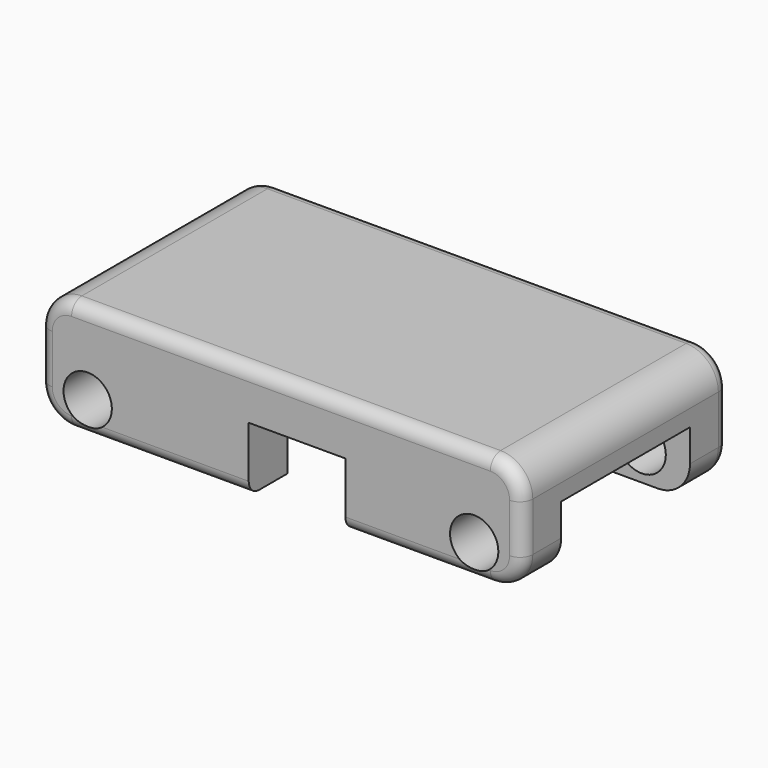
from build123d import *

# Parameters (mm, degrees)
F0_R          = 4.7625
F1_DEPTH      = 25.4
F2_W          = 31.75
F2_H          = 12.7
F3_DEPTH      = 47.626
F3_DEPTH_BACK = 47.626
F4_T1_DEPTH   = 82.55
F4_T3_DEPTH   = 9.6279704779
F4_T5_DEPTH   = 41.275
F4_T7_DEPTH   = 34.925
F4_T10_ANGLE  = 90
F4_T12_ANGLE  = 90
F4_T14_ANGLE  = 90
F4_T16_ANGLE  = 90
F4_T18_ANGLE  = 90
F4_T20_ANGLE  = 90
F4_T22_ANGLE  = 90
F4_T24_ANGLE  = 90


# Not quite as in the source:
# - a fillet or chamfer that OpenCascade refuses, or shapes differently, is made with other operations: its cross-section is extruded or revolved along the edge and cut away or added


with BuildPart() as f1:
    # F0 (on Front) → F1 (new body, symmetric)
    with BuildSketch(Plane.XZ):
        with BuildLine():
            Line((41.275, 15.9779704779), (-41.275, 15.9779704779))
            ThreePointArc((-41.275, 15.9779704779), (-45.7651280605, 14.1180985385), (-47.625, 9.6279704779))
            Line((-47.625, 9.6279704779), (-47.625, 0))
            ThreePointArc((-47.625, 0), (-45.7651280605, -4.4901280605), (-41.275, -6.35))
            Line((-41.275, -6.35), (-6.35, -6.35))
            Line((-6.35, -6.35), (-6.35, 6.35))
            Line((-6.35, 6.35), (12.7, 6.35))
            Line((12.7, 6.35), (12.7, -6.35))
            Line((12.7, -6.35), (41.275, -6.35))
            ThreePointArc((41.275, -6.35), (45.7651280605, -4.4901280605), (47.625, 0))
            Line((47.625, 0), (47.625, 9.6279704779))
            ThreePointArc((47.625, 9.6279704779), (45.7651280605, 14.1180985385), (41.275, 15.9779704779))
        make_face()
        with Locations((-38.1, 0)):
            Circle(F0_R, mode=Mode.SUBTRACT)
        with Locations((38.1, 0)):
            Circle(F0_R, mode=Mode.SUBTRACT)
    extrude(amount=F1_DEPTH, both=True)

    # F2 (on Right) → F3 (cut, two sides)
    with BuildSketch(Plane.YZ) as f3_sk:
        Rectangle(F2_W, F2_H)
    extrude(amount=F3_DEPTH, mode=Mode.SUBTRACT)
    extrude(f3_sk.sketch, amount=-F3_DEPTH_BACK, mode=Mode.SUBTRACT)

    # F4: fillet of radius 2.54 on 18 edges, made by hand

    # F4_s2 → F4_t1 (cut)
    with BuildSketch(Plane.YZ.offset(-41.275)):
        with BuildLine():
            ThreePointArc((22.86, 15.9779704779), (24.6560512242, 15.2340217022), (25.4, 13.4379704779))
            Line((25.4, 13.4379704779), (25.4, 15.9779704779))
            Line((25.4, 15.9779704779), (22.86, 15.9779704779))
        make_face()
        with BuildLine():
            ThreePointArc((-22.86, 15.9779704779), (-24.6560512242, 15.2340217022), (-25.4, 13.4379704779))
            Line((-25.4, 13.4379704779), (-25.4, 15.9779704779))
            Line((-25.4, 15.9779704779), (-22.86, 15.9779704779))
        make_face()
    extrude(amount=F4_T1_DEPTH, mode=Mode.SUBTRACT)

    # F4_s4 → F4_t3 (cut)
    with BuildSketch(Plane.XY):
        with BuildLine():
            ThreePointArc((-45.085, 25.4), (-46.8810512242, 24.6560512242), (-47.625, 22.86))
            Line((-47.625, 22.86), (-47.625, 25.4))
            Line((-47.625, 25.4), (-45.085, 25.4))
        make_face()
        with BuildLine():
            ThreePointArc((45.085, 25.4), (46.8810512242, 24.6560512242), (47.625, 22.86))
            Line((47.625, 22.86), (47.625, 25.4))
            Line((47.625, 25.4), (45.085, 25.4))
        make_face()
        with BuildLine():
            ThreePointArc((-45.085, -25.4), (-46.8810512242, -24.6560512242), (-47.625, -22.86))
            Line((-47.625, -22.86), (-47.625, -25.4))
            Line((-47.625, -25.4), (-45.085, -25.4))
        make_face()
        with BuildLine():
            ThreePointArc((45.085, -25.4), (46.8810512242, -24.6560512242), (47.625, -22.86))
            Line((47.625, -22.86), (47.625, -25.4))
            Line((47.625, -25.4), (45.085, -25.4))
        make_face()
    extrude(amount=F4_T3_DEPTH, mode=Mode.SUBTRACT)

    # F4_s6 → F4_t5 (cut)
    with BuildSketch(Plane.YZ.offset(-41.275)):
        with BuildLine():
            ThreePointArc((25.4, -3.81), (24.6560512242, -5.6060512242), (22.86, -6.35))
            Line((22.86, -6.35), (25.4, -6.35))
            Line((25.4, -6.35), (25.4, -3.81))
        make_face()
        with BuildLine():
            ThreePointArc((-25.4, -3.81), (-24.6560512242, -5.6060512242), (-22.86, -6.35))
            Line((-22.86, -6.35), (-25.4, -6.35))
            Line((-25.4, -6.35), (-25.4, -3.81))
        make_face()
    extrude(amount=F4_T5_DEPTH, mode=Mode.SUBTRACT)

    # F4_s8 → F4_t7 (cut)
    with BuildSketch(Plane.YZ.offset(6.35)):
        with BuildLine():
            ThreePointArc((25.4, -3.81), (24.6560512242, -5.6060512242), (22.86, -6.35))
            Line((22.86, -6.35), (25.4, -6.35))
            Line((25.4, -6.35), (25.4, -3.81))
        make_face()
        with BuildLine():
            ThreePointArc((-25.4, -3.81), (-24.6560512242, -5.6060512242), (-22.86, -6.35))
            Line((-22.86, -6.35), (-25.4, -6.35))
            Line((-25.4, -6.35), (-25.4, -3.81))
        make_face()
    extrude(amount=F4_T7_DEPTH, mode=Mode.SUBTRACT)

    # F4_s9 → F4_t10 (revolve, cut)
    with BuildSketch(Plane.YZ.offset(-41.275)):
        with BuildLine():
            ThreePointArc((25.4, 13.4379704779), (24.6560512242, 15.2340217022), (22.86, 15.9779704779))
            Line((22.86, 15.9779704779), (25.4, 15.9779704779))
            Line((25.4, 15.9779704779), (25.4, 13.4379704779))
        make_face()
    revolve(axis=Axis((-41.275, 25.4, 9.6279704779), (0, -1, 0)), revolution_arc=F4_T10_ANGLE, mode=Mode.SUBTRACT)

    # F4_s11 → F4_t12 (revolve, cut)
    with BuildSketch(Plane.XY):
        with BuildLine():
            ThreePointArc((-45.085, 25.4), (-46.8810512242, 24.6560512242), (-47.625, 22.86))
            Line((-47.625, 22.86), (-47.625, 25.4))
            Line((-47.625, 25.4), (-45.085, 25.4))
        make_face()
    revolve(axis=Axis((-41.275, 25.4, 0), (0, -1, 0)), revolution_arc=F4_T12_ANGLE, mode=Mode.SUBTRACT)

    # F4_s13 → F4_t14 (revolve, cut)
    with BuildSketch(Plane.YZ.offset(41.275)):
        with BuildLine():
            ThreePointArc((25.4, -3.81), (24.6560512242, -5.6060512242), (22.86, -6.35))
            Line((22.86, -6.35), (25.4, -6.35))
            Line((25.4, -6.35), (25.4, -3.81))
        make_face()
    revolve(axis=Axis((41.275, 25.4, 0), (0, -1, 0)), revolution_arc=F4_T14_ANGLE, mode=Mode.SUBTRACT)

    # F4_s15 → F4_t16 (revolve, cut)
    with BuildSketch(Plane.XY.offset(9.6279704779)):
        with BuildLine():
            ThreePointArc((45.085, 25.4), (46.8810512242, 24.6560512242), (47.625, 22.86))
            Line((47.625, 22.86), (47.625, 25.4))
            Line((47.625, 25.4), (45.085, 25.4))
        make_face()
    revolve(axis=Axis((41.275, 25.4, 9.6279704779), (0, -1, 0)), revolution_arc=F4_T16_ANGLE, mode=Mode.SUBTRACT)

    # F4_s17 → F4_t18 (revolve, cut)
    with BuildSketch(Plane.YZ.offset(-41.275)):
        with BuildLine():
            ThreePointArc((-22.86, 15.9779704779), (-24.6560512242, 15.2340217022), (-25.4, 13.4379704779))
            Line((-25.4, 13.4379704779), (-25.4, 15.9779704779))
            Line((-25.4, 15.9779704779), (-22.86, 15.9779704779))
        make_face()
    revolve(axis=Axis((-41.275, -25.4, 9.6279704779), (0, -1, 0)), revolution_arc=F4_T18_ANGLE, mode=Mode.SUBTRACT)

    # F4_s19 → F4_t20 (revolve, cut)
    with BuildSketch(Plane.XY):
        with BuildLine():
            ThreePointArc((-45.085, -25.4), (-46.8810512242, -24.6560512242), (-47.625, -22.86))
            Line((-47.625, -22.86), (-47.625, -25.4))
            Line((-47.625, -25.4), (-45.085, -25.4))
        make_face()
    revolve(axis=Axis((-41.275, -25.4, 0), (0, -1, 0)), revolution_arc=F4_T20_ANGLE, mode=Mode.SUBTRACT)

    # F4_s21 → F4_t22 (revolve, cut)
    with BuildSketch(Plane.YZ.offset(41.275)):
        with BuildLine():
            ThreePointArc((-25.4, -3.81), (-24.6560512242, -5.6060512242), (-22.86, -6.35))
            Line((-22.86, -6.35), (-25.4, -6.35))
            Line((-25.4, -6.35), (-25.4, -3.81))
        make_face()
    revolve(axis=Axis((41.275, -25.4, 0), (0, -1, 0)), revolution_arc=F4_T22_ANGLE, mode=Mode.SUBTRACT)

    # F4_s23 → F4_t24 (revolve, cut)
    with BuildSketch(Plane.XY.offset(9.6279704779)):
        with BuildLine():
            ThreePointArc((45.085, -25.4), (46.8810512242, -24.6560512242), (47.625, -22.86))
            Line((47.625, -22.86), (47.625, -25.4))
            Line((47.625, -25.4), (45.085, -25.4))
        make_face()
    revolve(axis=Axis((41.275, -25.4, 9.6279704779), (0, -1, 0)), revolution_arc=F4_T24_ANGLE, mode=Mode.SUBTRACT)


solid = f1.part
